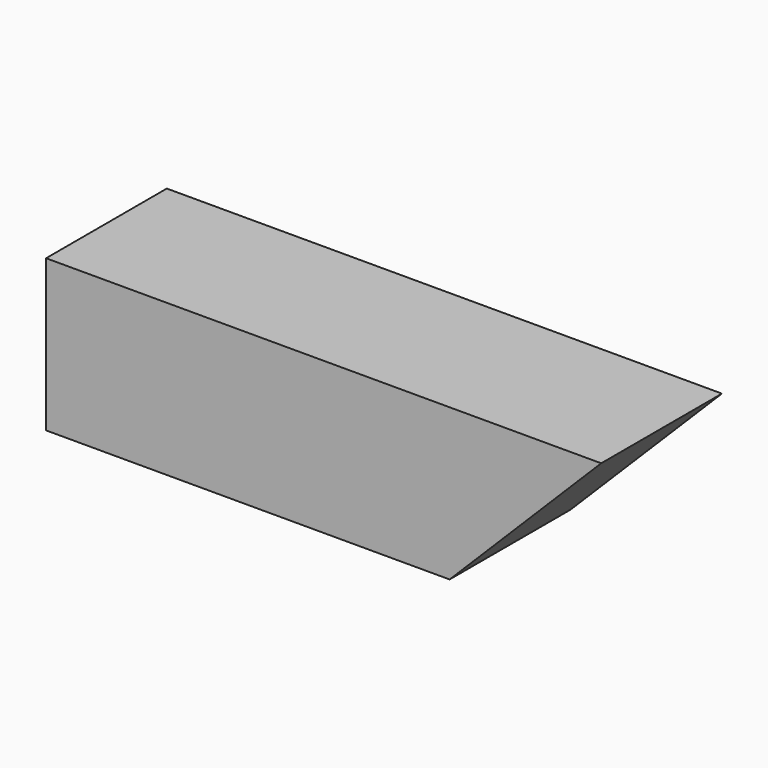
from build123d import *

# Parameters (mm, degrees)
F0_W     = 104.648
F0_H     = 28.448
F1_DEPTH = 28.575
F2_SIZE2 = 28.57499
F2_SIZE  = 28.57499


# Not quite as in the source:
# - a fillet or chamfer is up to 0.001 mm smaller than in the source, because OpenCascade refuses the exact size


with BuildPart() as f1:
    # F0 (on Top) → F1 (new body)
    with BuildSketch(Plane.XY):
        with Locations((-25.6716595031, -3.0957325469)):
            Rectangle(F0_W, F0_H)
    extrude(amount=F1_DEPTH)

    # F2 (size 28.575 and 28.575 in the source; OpenCascade refuses exactly that, so slightly less here)
    f2_edges = [f1.edges().sort_by_distance(p)[0] for p in [
        (26.65234, -3.095733, 0),
    ]]
    chamfer(f2_edges, length=F2_SIZE, length2=F2_SIZE2)


solid = f1.part
